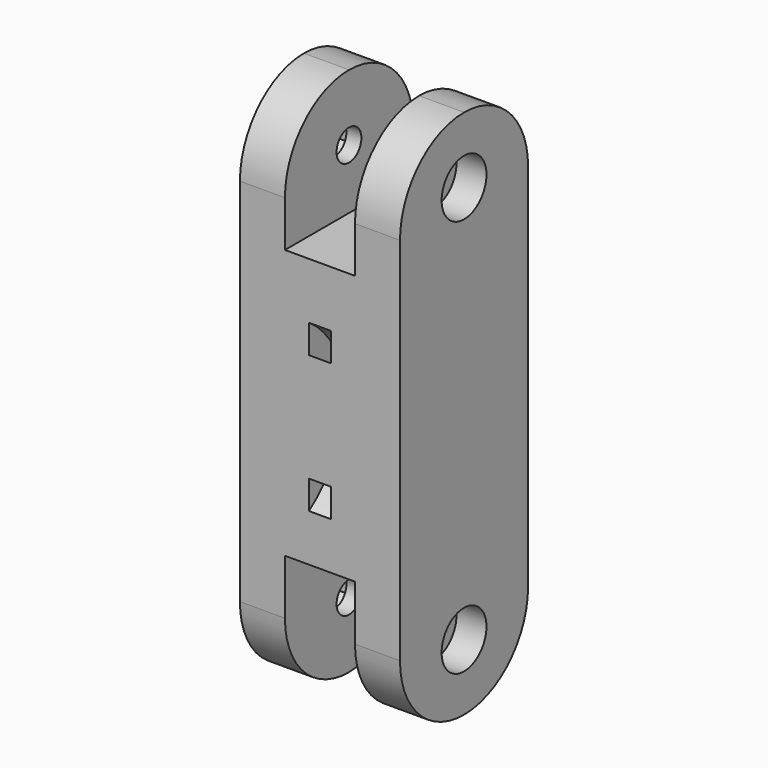
from build123d import *

# Parameters (mm, degrees)
F1_DEPTH  = 16
F2_R      = 7.99999
F3_R      = 1.55
F4_DEPTH  = 12.5
F5_DEPTH  = 25
F6_R      = 2.8
F7_DEPTH  = 3
F9_DEPTH  = 3
F10_R     = 1.125
F12_R     = 1.125
F15_DEPTH = 12.5
F17_DEPTH = 1.1


# Not quite as in the source:
# - a fillet or chamfer is up to 0.001 mm smaller than in the source, because OpenCascade refuses the exact size


with BuildPart() as f1:
    # F0 (on Front) → F1 (new body)
    with BuildSketch(Plane.XZ):
        Polygon((8, -18), (8, 18), (8, 26.5), (3.5, 26.5), (3.5, 13.9081878588), (-3.5, 13.9081878588), (-3.5, 26.5), (-8, 26.5), (-8, 18), (-8, -18), (-8, -26.5), (-3.5, -26.5), (-3.5, -18), (-3.5, -13), (3.5, -13), (3.5, -18), (3.5, -26.5), (8, -26.5), align=None)
    extrude(amount=F1_DEPTH)

    # F2 (radius 8 in the source; OpenCascade refuses exactly that, so slightly less here)
    f2_edges = [f1.edges().sort_by_distance(p)[0] for p in [
        (5.75, -16, 26.5),
        (-5.75, -16, 26.5),
        (-5.75, 0, 26.5),
        (5.75, 0, 26.5),
        (5.75, -16, -26.5),
        (-5.75, -16, -26.5),
        (5.75, 0, -26.5),
        (-5.75, 0, -26.5),
    ]]
    fillet(f2_edges, radius=F2_R)

    # F3 (on face) → F4 (cut, symmetric)
    with BuildSketch(Plane.YZ.offset(8)):
        with Locations((-8, 19.8896080256)):
            Circle(F3_R)
        with Locations((-8, -19.8896080256)):
            Circle(F3_R)
    extrude(amount=F4_DEPTH, both=True, mode=Mode.SUBTRACT)

    # F3 (on face) → F5 (cut)
    with BuildSketch(Plane.YZ.offset(8)):
        with Locations((-8, 19.8896080256)):
            Circle(F3_R)
        with Locations((-8, -19.8896080256)):
            Circle(F3_R)
    extrude(amount=-F5_DEPTH, mode=Mode.SUBTRACT)

    # F6 (on face) → F7 (cut)
    with BuildSketch(Plane.YZ.offset(8)):
        with Locations((-8, 19.8896080256)):
            Circle(F6_R)
        with Locations((-8, -19.8896080256)):
            Circle(F6_R)
    extrude(amount=-F7_DEPTH, mode=Mode.SUBTRACT)

    # F8 (on face) → F9 (cut)
    with BuildSketch(Plane(origin=(-8, 0, 0), x_dir=(0, -1, 0), z_dir=(-1, 0, 0))):
        Polygon((10.75, 18.3018947853), (10.75, 21.4773212658), (8, 23.0650345061), (5.25, 21.4773212658), (5.25, 18.3018947853), (8, 16.714181545), align=None)
        Polygon((5.25, -18.3018947853), (5.25, -21.4773212658), (8, -23.0650345061), (10.75, -21.4773212658), (10.75, -18.3018947853), (8, -16.714181545), align=None)
    extrude(amount=-F9_DEPTH, mode=Mode.SUBTRACT)

    # F10 (on face) → F11 (revolve)
    with BuildSketch(Plane.XZ.offset(16)):
        with Locations((-3, 0)):
            Circle(F10_R)
    revolve(axis=Axis((0, -16, 0.0619328348), (0, 0, -1)))

    # F12 (on face) → F13 (revolve)
    with BuildSketch(Plane(origin=(0, 0, 0), x_dir=(-1, 0, 0), z_dir=(0, 1, 0))):
        with Locations((3, 0)):
            Circle(F12_R)
    revolve(axis=Axis((0, 0, 0.5132202059), (0, 0, -1)))

    # F14 (on Top) → F15 (cut, symmetric)
    with BuildSketch(Plane.XY):
        Polygon((1.875, -16), (-1.875, -16), (-4.125, -16), (-8, -16), (-8, -21.5492993593), (8, -21.5492993593), (8, -16), (4.125, -16), align=None)
    extrude(amount=F15_DEPTH, both=True, mode=Mode.SUBTRACT)

    # F16 (on Right) → F17 (cut, symmetric)
    with BuildSketch(Plane.YZ):
        with BuildLine():
            Line((-16, -5.4295487842), (-16, -8.2849260709))
            ThreePointArc((-16, -8.2849260709), (-11.6, 0), (-16, 8.2849260709))
            Line((-16, 8.2849260709), (-16, 5.4295487842))
            ThreePointArc((-16, 5.4295487842), (-13.8, 0), (-16, -5.4295487842))
        make_face()
    extrude(amount=F17_DEPTH, both=True, mode=Mode.SUBTRACT)


solid = f1.part
